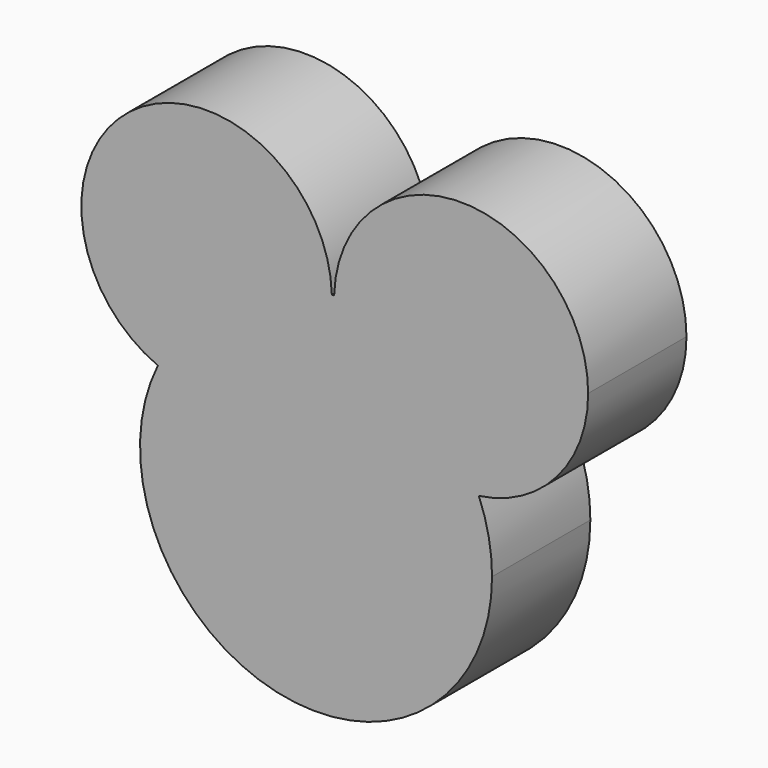
from build123d import *

# Parameters (mm, degrees)
F1_DEPTH = 25.4


with BuildPart() as f1:
    # F0 (on Front) → F1 (new body)
    with BuildSketch(Plane.XZ):
        with BuildLine():
            ThreePointArc((-37.2795093382, 40.0635529992), (-37.0944265378, 41.8428324334), (-37.0326339638, 43.6306446791))
            ThreePointArc((-37.0326339638, 43.6306446791), (-37.0352597257, 43.9993926792), (-37.0431364787, 44.3680658937))
            Line((-37.0431364787, 44.3680658937), (-59.2393539846, 44.3680658937))
            Line((-59.2393539846, 44.3680658937), (-59.2393539846, 34.8789981649))
            ThreePointArc((-59.2393539846, 34.8789981649), (-48.6715325086, 39.2167813917), (-37.2795093382, 40.0635529992))
        make_face()
        with BuildLine():
            ThreePointArc((-37.0431364787, 44.3680658937), (-37.0352597257, 43.9993926792), (-37.0326339638, 43.6306446791))
            ThreePointArc((-37.0326339638, 43.6306446791), (-37.0944265378, 41.8428324334), (-37.2795093382, 40.0635529992))
            ThreePointArc((-37.2795093382, 40.0635529992), (-36.8032339812, 40.0205567646), (-36.3275649384, 39.9713038099))
            ThreePointArc((-36.3275649384, 39.9713038099), (-36.5428213794, 42.1645221032), (-36.573424985, 44.3680658936))
            Line((-36.573424985, 44.3680658937), (-37.0431364787, 44.3680658937))
        make_face()
        with BuildLine():
            Line((-59.2393539846, 44.3680658937), (-37.0431364787, 44.3680658937))
            ThreePointArc((-37.0431364787, 44.3680658937), (-77.5434180545, 65.0043168763), (-73.0012082171, 19.7771569817))
            ThreePointArc((-73.0012082171, 19.7771569817), (-67.2022274173, 28.3140227514), (-59.2393539846, 34.8789981649))
            Line((-59.2393539846, 34.8789981649), (-59.2393539846, 44.3680658937))
        make_face()
        with BuildLine():
            ThreePointArc((-36.3275649384, 39.9713038099), (-36.8032339812, 40.0205567646), (-37.2795093382, 40.0635529992))
            ThreePointArc((-37.2795093382, 40.0635529992), (-44.4588292576, 25.4802541483), (-58.915556877, 18.0493547131))
            Line((-58.915556877, 18.0493547131), (-16.2551814161, 18.0493547131))
            ThreePointArc((-16.2551814161, 18.0493547131), (-29.6914752573, 25.897095458), (-36.3275649384, 39.9713038099))
        make_face()
        with BuildLine():
            ThreePointArc((-58.915556877, 18.0493547131), (-44.4588292576, 25.4802541483), (-37.2795093382, 40.0635529992))
            ThreePointArc((-37.2795093382, 40.0635529992), (-48.6715325086, 39.2167813917), (-59.2393539846, 34.8789981649))
            Line((-59.2393539846, 34.8789981649), (-59.2393539846, 18.0493547131))
            Line((-59.2393539846, 18.0493547131), (-58.915556877, 18.0493547131))
        make_face()
        with BuildLine():
            ThreePointArc((-59.2393539846, 34.8789981649), (-67.2022274173, 28.3140227514), (-73.0012082171, 19.7771569817))
            ThreePointArc((-73.0012082171, 19.7771569817), (-66.0790584232, 17.9294636931), (-58.915556877, 18.0493547131))
            Line((-58.915556877, 18.0493547131), (-59.2393539846, 18.0493547131))
            Line((-59.2393539846, 18.0493547131), (-59.2393539846, 34.8789981649))
        make_face()
        with BuildLine():
            ThreePointArc((-58.915556877, 18.0493547131), (-66.0790584232, 17.9294636931), (-73.0012082171, 19.7771569817))
            ThreePointArc((-73.0012082171, 19.7771569817), (-48.5063899421, -31.6353638875), (-3.9320745419, 3.8100001402))
            ThreePointArc((-3.9320745419, 3.8100001402), (-4.620150317, 10.8521017976), (-6.6583498303, 17.6278221851))
            ThreePointArc((-6.6583498303, 17.6278221851), (-11.4762045796, 17.3960309275), (-16.2551814161, 18.0493547131))
            Line((-16.2551814161, 18.0493547131), (-58.915556877, 18.0493547131))
        make_face()
        with BuildLine():
            Line((-16.2551814161, 44.3680658937), (-36.573424985, 44.3680658937))
            ThreePointArc((-36.573424985, 44.3680658936), (-36.5428213794, 42.1645221032), (-36.3275649384, 39.9713038099))
            ThreePointArc((-36.3275649384, 39.9713038099), (-25.6065541108, 37.085516119), (-16.2551814161, 31.1005622773))
            Line((-16.2551814161, 31.1005622773), (-16.2551814161, 44.3680658937))
        make_face()
        with BuildLine():
            ThreePointArc((15.9360373073, 43.6306446791), (-9.9551248939, 69.8879647074), (-36.573424985, 44.3680658936))
            Line((-36.573424985, 44.3680658937), (-16.2551814161, 44.3680658937))
            Line((-16.2551814161, 44.3680658937), (-16.2551814161, 31.1005622773))
            ThreePointArc((-16.2551814161, 31.1005622773), (-10.6808873976, 24.916861741), (-6.6583498303, 17.6278221851))
            ThreePointArc((-6.6583498303, 17.6278221851), (9.4983266183, 26.4067288367), (15.9360373073, 43.6306446791))
        make_face()
        with BuildLine():
            ThreePointArc((-16.2551814161, 31.1005622773), (-25.6065541108, 37.085516119), (-36.3275649384, 39.9713038099))
            ThreePointArc((-36.3275649384, 39.9713038099), (-29.6914752573, 25.897095458), (-16.2551814161, 18.0493547131))
            Line((-16.2551814161, 18.0493547131), (-16.2551814161, 31.1005622773))
        make_face()
        with BuildLine():
            Line((-16.2551814161, 31.1005622773), (-16.2551814161, 18.0493547131))
            ThreePointArc((-16.2551814161, 18.0493547131), (-11.4762045796, 17.3960309275), (-6.6583498303, 17.6278221851))
            ThreePointArc((-6.6583498303, 17.6278221851), (-10.6808873976, 24.916861741), (-16.2551814161, 31.1005622773))
        make_face()
    extrude(amount=F1_DEPTH)


solid = f1.part
